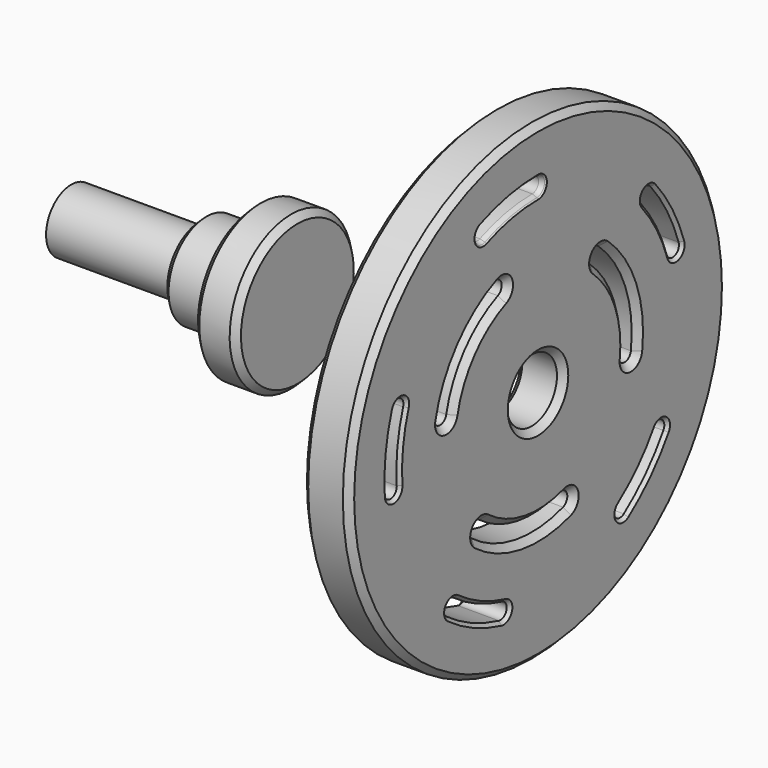
from build123d import *

# Parameters (mm, degrees)
F0_R         = 75
F0_R_2       = 10
F1_DEPTH     = 15
F2_SIZE      = 2
F4_DEPTH     = 15.001
F5_SIZE      = 1
F6_SIZE      = 2
F8_DEPTH     = 15.001
F9_T2_ANGLE  = 55.3680606349
F9_T4_ANGLE  = 22.2231670965
F9_T6_ANGLE  = 55.3680606349
F9_T8_ANGLE  = 55.3680606349
F9_T10_ANGLE = 55.3680606349
F9_T12_ANGLE = 180
F9_T14_ANGLE = 180
F9_T16_ANGLE = 55.3680606349
F9_T18_ANGLE = 180
F9_T20_ANGLE = 180
F9_T22_ANGLE = 55.3680606349
F9_T24_ANGLE = 180
F9_T26_ANGLE = 180
F9_T28_ANGLE = 55.3680606349
F9_T30_ANGLE = 180
F9_T32_ANGLE = 180
F9_T34_ANGLE = 22.2231670965
F9_T36_ANGLE = 180
F9_T38_ANGLE = 180
F9_T40_ANGLE = 55.3680606349
F12_SIZE     = 2


# Not quite as in the source:
# - a fillet or chamfer that OpenCascade refuses, or shapes differently, is made with other operations: its cross-section is extruded or revolved along the edge and cut away or added
# - a feature names something its author has since deleted; it is built from what else it names


with BuildPart() as f1:
    # F0 (on Right) → F1 (new body)
    with BuildSketch(Plane.YZ):
        Circle(F0_R)
        Circle(F0_R_2, mode=Mode.SUBTRACT)
    extrude(amount=F1_DEPTH)

    # F2
    f2_edges = [f1.edges().sort_by_distance(p)[0] for p in [
        (15, -75, 0),
        (0, -75, 0),
        (15, -10, 0),
    ]]
    chamfer(f2_edges, length=F2_SIZE)

    # F3 (on face) → F4 (cut, through all)
    with BuildSketch(Plane.YZ.offset(15)):
        with BuildLine():
            ThreePointArc((0, 55), (2.5, 57.5), (0, 60))
            ThreePointArc((0, 60), (-11.5632210939, 58.8752232941), (-22.6929074633, 55.5430639312))
            ThreePointArc((-22.6929074633, 55.5430639312), (-24.0616639828, 52.2832317897), (-20.8018318414, 50.9144752702))
            ThreePointArc((-20.8018318414, 50.9144752702), (-10.599619336, 53.9689546863), (0, 55))
        make_face()
        with BuildLine():
            ThreePointArc((57.0633909777, 18.5410196625), (52.4204329345, 29.1907213162), (45.8120988288, 38.7459881911))
            ThreePointArc((45.8120988288, 38.7459881911), (42.2888452029, 39.0404094676), (41.9944239264, 35.5171558418))
            ThreePointArc((41.9944239264, 35.5171558418), (48.0520635233, 26.7581612065), (52.3081083962, 16.9959346906))
            ThreePointArc((52.3081083962, 16.9959346906), (55.4582921729, 15.3908358858), (57.0633909777, 18.5410196625))
        make_face()
        with BuildLine():
            ThreePointArc((35.2671151375, -48.5410196625), (43.9608303524, -40.8343653646), (51.0063416355, -31.5967263014))
            ThreePointArc((51.0063416355, -31.5967263014), (50.1976076632, -28.154931804), (46.7558131659, -28.9636657763))
            ThreePointArc((46.7558131659, -28.9636657763), (40.297427823, -37.4315015842), (32.3281888761, -44.4959346906))
            ThreePointArc((32.3281888761, -44.4959346906), (31.7751095209, -47.9879403073), (35.2671151375, -48.5410196625))
        make_face()
        with BuildLine():
            ThreePointArc((-35.2671151375, -48.5410196625), (-25.2511456031, -54.4277470205), (-14.2884460563, -58.2738389785))
            ThreePointArc((-14.2884460563, -58.2738389785), (-11.2650175131, -56.4411142735), (-13.0977422182, -53.4176857303))
            ThreePointArc((-13.0977422182, -53.4176857303), (-23.1468834695, -49.8921014355), (-32.3281888761, -44.4959346906))
            ThreePointArc((-32.3281888761, -44.4959346906), (-35.8201944928, -45.0490140458), (-35.2671151375, -48.5410196625))
        make_face()
        with BuildLine():
            ThreePointArc((-57.0633909777, 18.5410196625), (-59.5668965899, 7.1961677748), (-59.8370869447, -4.4184868423))
            ThreePointArc((-59.8370869447, -4.4184868423), (-57.1597713702, -6.7275951799), (-54.8506630326, -4.0502796055))
            ThreePointArc((-54.8506630326, -4.0502796055), (-54.6029885408, 6.5964871269), (-52.3081083962, 16.9959346906))
            ThreePointArc((-52.3081083962, 16.9959346906), (-53.913207201, 20.1461184673), (-57.0633909777, 18.5410196625))
        make_face()
    extrude(amount=-F4_DEPTH, mode=Mode.SUBTRACT)

    # F5
    f5_edges = [f1.edges().sort_by_distance(p)[0] for p in [
        (15, -10.599619, 53.968955),
        (15, -54.602989, 6.596487),
        (15, 48.052064, 26.758161),
        (15, 40.297428, -37.431502),
        (15, -23.146883, -49.892101),
        (0, -10.599619, 53.968955),
        (0, -54.602989, 6.596487),
        (0, -23.146883, -49.892101),
        (0, 40.297428, -37.431502),
        (0, 48.052064, 26.758161),
        (0, -35.820194, -45.049014),
        (0, -25.251146, -54.427747),
        (0, -11.265018, -56.441114),
        (0, 43.96083, -40.834365),
        (0, 50.197608, -28.154932),
        (0, 31.77511, -47.98794),
        (0, -53.913207, 20.146118),
        (0, -59.566897, 7.196168),
        (0, -57.159771, -6.727595),
        (0, 2.5, 57.5),
        (0, -11.563221, 58.875223),
        (0, -24.061664, 52.283232),
        (0, 55.458292, 15.390836),
        (0, 52.420433, 29.190721),
        (0, 42.288845, 39.040409),
        (15, -35.820194, -45.049014),
        (15, -25.251146, -54.427747),
        (15, -11.265018, -56.441114),
        (15, 43.96083, -40.834365),
        (15, 50.197608, -28.154932),
        (15, 31.77511, -47.98794),
        (15, -53.913207, 20.146118),
        (15, -59.566897, 7.196168),
        (15, -57.159771, -6.727595),
        (15, 55.458292, 15.390836),
        (15, 52.420433, 29.190721),
        (15, 42.288845, 39.040409),
    ]]
    chamfer(f5_edges, length=F5_SIZE)

    # F6
    f6_edges = [f1.edges().sort_by_distance(p)[0] for p in [
        (0, -10, 0),
    ]]
    chamfer(f6_edges, length=F6_SIZE)

    # F7 (on face) → F8 (cut, through all)
    with BuildSketch(Plane(origin=(0, 0, 0), x_dir=(0, -1, 0), z_dir=(-1, 0, 0))):
        with BuildLine():
            ThreePointArc((33.9430104886, 7.0805472984), (36.9008441725, 5.1437406745), (38.8376507964, 8.1015743584))
            ThreePointArc((38.8376507964, 8.1015743584), (30.6276860735, 25.2179196654), (15.4053995333, 36.5605291494))
            ThreePointArc((15.4053995333, 36.5605291494), (12.1308125803, 35.2274574006), (13.4638843291, 31.9528704476))
            ThreePointArc((13.4638843291, 31.9528704476), (26.7677330713, 22.0397499373), (33.9430104886, 7.0805472984))
        make_face()
        with BuildLine():
            ThreePointArc((-10.8395714112, -32.9357830132), (-13.9958119916, -34.5289388117), (-12.4026561931, -37.6851793922))
            ThreePointArc((-12.4026561931, -37.6851793922), (6.5255160241, -39.1333140315), (23.9596472526, -31.621731926))
            ThreePointArc((23.9596472526, -31.621731926), (24.4424667295, -28.1193205634), (20.9400553669, -27.6365010865))
            ThreePointArc((20.9400553669, -27.6365010865), (5.7031168031, -34.2014118101), (-10.8395714112, -32.9357830132))
        make_face()
        with BuildLine():
            ThreePointArc((-23.1034390774, 25.8552357148), (-22.9050321809, 29.3851981372), (-26.4349946032, 29.5836050337))
            ThreePointArc((-26.4349946032, 29.5836050337), (-37.1532020976, 13.915394366), (-39.3650467858, -4.9387972235))
            ThreePointArc((-39.3650467858, -4.9387972235), (-36.5732793098, -7.1081368372), (-34.4039396961, -4.3163693612))
            ThreePointArc((-34.4039396961, -4.3163693612), (-32.4708498744, 12.1616618728), (-23.1034390774, 25.8552357148))
        make_face()
    extrude(amount=-F8_DEPTH, mode=Mode.SUBTRACT)

    # F9: chamfer of 2 on 5 edges, made by hand

    # F9_s1 → F9_t2 (revolve, cut)
    with BuildSketch(Plane(origin=(0, 0, 0), x_dir=(1, 0, 0), z_dir=(0, -0.204205412, -0.9789280616))):
        Polygon((13, 34.6736515393), (15, 32.6736515393), (15, 34.6736515393), align=None)
    revolve(axis=Axis((15, 0, 0), (-1, 0, 0)), revolution_arc=F9_T2_ANGLE, mode=Mode.SUBTRACT)

    # F9_s3 → F9_t4 (revolve, cut)
    with BuildSketch(Plane(origin=(0, 0, 0), x_dir=(1, 0, 0), z_dir=(0, -0.9257177322, -0.3782151244))):
        Polygon((13.1715728753, 55), (14.5857864376, 54.4142135624), (14, 55), align=None)
    revolve(axis=Axis((14, 0, 0), (-1, 0, 0)), revolution_arc=F9_T4_ANGLE, mode=Mode.SUBTRACT)

    # F9_s5 → F9_t6 (revolve, cut)
    with BuildSketch(Plane(origin=(0, 0, 0), x_dir=(1, 0, 0), z_dir=(0, -0.7456738638, 0.6663111052))):
        Polygon((13, 34.6736515393), (15, 32.6736515393), (15, 34.6736515393), align=None)
    revolve(axis=Axis((15, 0, 0), (-1, 0, 0)), revolution_arc=F9_T6_ANGLE, mode=Mode.SUBTRACT)

    # F9_s7 → F9_t8 (revolve, cut)
    with BuildSketch(Plane(origin=(0, 0, 0), x_dir=(1, 0, 0), z_dir=(0, -0.7970461679, 0.6039183771))):
        Polygon((0, -32.6736515393), (2, -34.6736515393), (0, -34.6736515393), align=None)
    revolve(axis=Axis((0, 0, 0), (1, 0, 0)), revolution_arc=F9_T8_ANGLE, mode=Mode.SUBTRACT)

    # F9_s9 → F9_t10 (revolve, cut)
    with BuildSketch(Plane(origin=(0, 0, 0), x_dir=(1, 0, 0), z_dir=(0, 0.9498792758, 0.3126169564))):
        Polygon((13, 34.6736515393), (15, 32.6736515393), (15, 34.6736515393), align=None)
    revolve(axis=Axis((15, 0, 0), (-1, 0, 0)), revolution_arc=F9_T10_ANGLE, mode=Mode.SUBTRACT)

    # F9_s11 → F9_t12 (revolve, cut)
    with BuildSketch(Plane(origin=(0, 0, 0), x_dir=(1, 0, 0), z_dir=(0, -0.9498792758, -0.3126169564))):
        Polygon((13, -34.6736515393), (15, -32.6736515393), (15, -34.6736515393), align=None)
    revolve(axis=Axis((15, 11.6211138021, -35.3104812027), (-1, 0, 0)), revolution_arc=F9_T12_ANGLE, mode=Mode.SUBTRACT)

    # F9_s13 → F9_t14 (revolve, cut)
    with BuildSketch(Plane(origin=(0, 0, 0), x_dir=(1, 0, 0), z_dir=(0, 0.7970461679, -0.6039183771))):
        Polygon((13, 39.6736515393), (15, 41.6736515393), (15, 39.6736515393), align=None)
    revolve(axis=Axis((15, -22.4498513097, -29.6291165062), (-1, 0, 0)), revolution_arc=F9_T14_ANGLE, mode=Mode.SUBTRACT)

    # F9_s15 → F9_t16 (revolve, cut)
    with BuildSketch(Plane(origin=(0, 0, 0), x_dir=(1, 0, 0), z_dir=(0, 0.9498792758, 0.3126169564))):
        Polygon((13, 39.6736515393), (15, 41.6736515393), (15, 39.6736515393), align=None)
    revolve(axis=Axis((15, 0, 0), (-1, 0, 0)), revolution_arc=F9_T16_ANGLE, mode=Mode.SUBTRACT)

    # F9_s17 → F9_t18 (revolve, cut)
    with BuildSketch(Plane(origin=(0, 0, 0), x_dir=(1, 0, 0), z_dir=(0, 0.7970461679, -0.6039183771))):
        Polygon((0, 41.6736515393), (2, 39.6736515393), (0, 39.6736515393), align=None)
    revolve(axis=Axis((0, -22.4498513097, -29.6291165062), (-1, 0, 0)), revolution_arc=F9_T18_ANGLE, mode=Mode.SUBTRACT)

    # F9_s19 → F9_t20 (revolve, cut)
    with BuildSketch(Plane(origin=(0, 0, 0), x_dir=(1, 0, 0), z_dir=(0, -0.9498792758, -0.3126169564))):
        Polygon((0, -32.6736515393), (2, -34.6736515393), (0, -34.6736515393), align=None)
    revolve(axis=Axis((0, 11.6211138021, -35.3104812027), (-1, 0, 0)), revolution_arc=F9_T20_ANGLE, mode=Mode.SUBTRACT)

    # F9_s21 → F9_t22 (revolve, cut)
    with BuildSketch(Plane(origin=(0, 0, 0), x_dir=(1, 0, 0), z_dir=(0, 0.9498792758, 0.3126169564))):
        Polygon((0, 41.6736515393), (2, 39.6736515393), (0, 39.6736515393), align=None)
    revolve(axis=Axis((0, 0, 0), (-1, 0, 0)), revolution_arc=F9_T22_ANGLE, mode=Mode.SUBTRACT)

    # F9_s23 → F9_t24 (revolve, cut)
    with BuildSketch(Plane(origin=(0, 0, 0), x_dir=(1, 0, 0), z_dir=(0, 0.7456738638, -0.6663111052))):
        Polygon((13, -34.6736515393), (15, -32.6736515393), (15, -34.6736515393), align=None)
    revolve(axis=Axis((15, 24.7692168403, 27.7194203743), (-1, 0, 0)), revolution_arc=F9_T24_ANGLE, mode=Mode.SUBTRACT)

    # F9_s25 → F9_t26 (revolve, cut)
    with BuildSketch(Plane(origin=(0, 0, 0), x_dir=(1, 0, 0), z_dir=(0, 0.1244855725, 0.992221418))):
        Polygon((13, 39.6736515393), (15, 41.6736515393), (15, 39.6736515393), align=None)
    revolve(axis=Axis((15, 36.8844932409, -4.6275832923), (-1, 0, 0)), revolution_arc=F9_T26_ANGLE, mode=Mode.SUBTRACT)

    # F9_s27 → F9_t28 (revolve, cut)
    with BuildSketch(Plane(origin=(0, 0, 0), x_dir=(1, 0, 0), z_dir=(0, -0.7456738638, 0.6663111052))):
        Polygon((13, 39.6736515393), (15, 41.6736515393), (15, 39.6736515393), align=None)
    revolve(axis=Axis((15, 0, 0), (-1, 0, 0)), revolution_arc=F9_T28_ANGLE, mode=Mode.SUBTRACT)

    # F9_s29 → F9_t30 (revolve, cut)
    with BuildSketch(Plane(origin=(0, 0, 0), x_dir=(1, 0, 0), z_dir=(0, 0.9257177322, 0.3782151244))):
        Polygon((13.1715728753, -60), (14.5857864376, -60.5857864376), (14, -60), align=None)
    revolve(axis=Axis((14, -21.7473696524, 53.2287696007), (1, 0, 0)), revolution_arc=F9_T30_ANGLE, mode=Mode.SUBTRACT)

    # F9_s31 → F9_t32 (revolve, cut)
    with BuildSketch(Plane.XZ):
        Polygon((13.1715728753, 55), (14.5857864376, 54.4142135624), (14, 55), align=None)
    revolve(axis=Axis((14, 0, 57.5), (1, 0, 0)), revolution_arc=F9_T32_ANGLE, mode=Mode.SUBTRACT)

    # F9_s33 → F9_t34 (revolve, cut)
    with BuildSketch(Plane.XZ):
        Polygon((13.1715728753, 60), (14.5857864376, 60.5857864376), (14, 60), align=None)
    revolve(axis=Axis((14, 0, 0), (1, 0, 0)), revolution_arc=F9_T34_ANGLE, mode=Mode.SUBTRACT)

    # F9_s35 → F9_t36 (revolve, cut)
    with BuildSketch(Plane(origin=(0, 0, 0), x_dir=(1, 0, 0), z_dir=(0, 0.204205412, 0.9789280616))):
        Polygon((13, -34.6736515393), (15, -32.6736515393), (15, -34.6736515393), align=None)
    revolve(axis=Axis((15, -36.3903306425, 7.5910608284), (-1, 0, 0)), revolution_arc=F9_T36_ANGLE, mode=Mode.SUBTRACT)

    # F9_s37 → F9_t38 (revolve, cut)
    with BuildSketch(Plane(origin=(0, 0, 0), x_dir=(1, 0, 0), z_dir=(0, -0.9215317404, -0.3883030408))):
        Polygon((13, 39.6736515393), (15, 41.6736515393), (15, 39.6736515393), align=None)
    revolve(axis=Axis((15, -14.4346419312, 34.2566997985), (-1, 0, 0)), revolution_arc=F9_T38_ANGLE, mode=Mode.SUBTRACT)

    # F9_s39 → F9_t40 (revolve, cut)
    with BuildSketch(Plane(origin=(0, 0, 0), x_dir=(1, 0, 0), z_dir=(0, -0.204205412, -0.9789280616))):
        Polygon((13, 39.6736515393), (15, 41.6736515393), (15, 39.6736515393), align=None)
    revolve(axis=Axis((15, 0, 0), (-1, 0, 0)), revolution_arc=F9_T40_ANGLE, mode=Mode.SUBTRACT)


with BuildPart() as f11:
    # F10 (on Front) → F11 (revolve)
    with BuildSketch(Plane.XZ):
        Polygon((-92.3496652881, 15), (-92.3496652881, 10), (-133.2587525919, 10), (-133.2587525919, 5), (-133.2587525919, 0), (-61.4405683377, 0), (-61.4405683377, 24.3939396538), (-75.0769336305, 24.3939396538), (-75.0769336305, 15), align=None)
    revolve(axis=Axis((-82.1223913184, 0, 0), (-1, 0, 0)))

    # F12
    f12_edges = [f11.edges().sort_by_distance(p)[0] for p in [
        (-92.349665, 0, -15),
        (-75.076934, 0, -24.39394),
        (-61.440568, 0, -24.39394),
    ]]
    chamfer(f12_edges, length=F12_SIZE)


solid = Compound([f1.part, f11.part])
